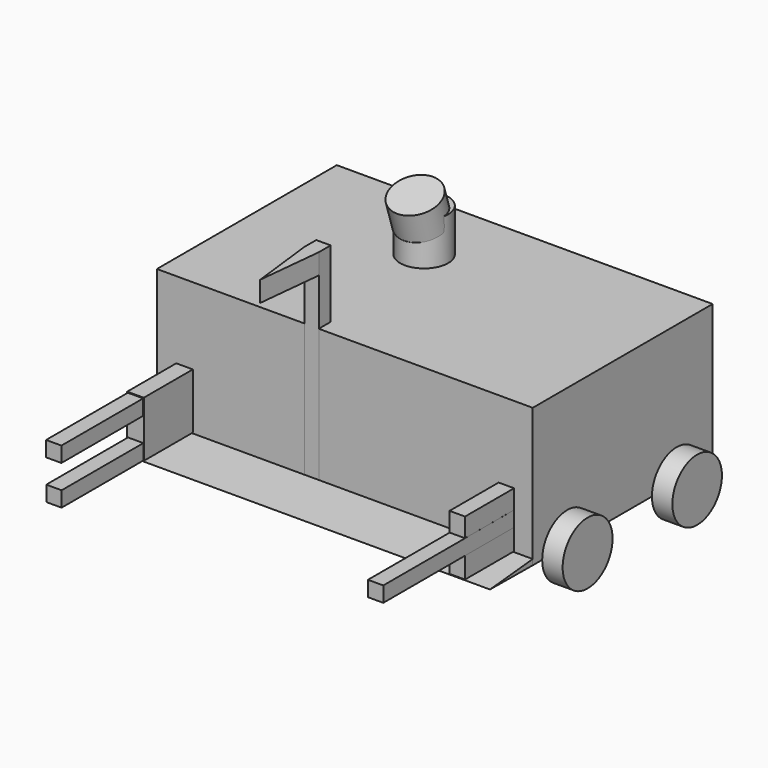
from build123d import *

# Parameters (mm, degrees)
F0_W      = 19.05
F0_H      = 19.05
F1_DEPTH  = 203.2
F2_W      = 20.5676518381
F2_H      = 69.0995454788
F3_DEPTH  = 76.2
F2_W_2    = 19.1925428808
F2_H_2    = 68.9241439104
F4_W      = 467.0027047396
F4_H      = 172.3322272301
F5_DEPTH  = 279.4
F6_R      = 38.6584580122
F7_DEPTH  = 19.05
F6_R_2    = 37.8719850625
F8_R      = 4.318122092
F9_DEPTH  = 26.924
F8_R_2    = 4.8859872563
F10_R     = 38.7883193787
F10_R_2   = 38.4875919081
F11_DEPTH = 25.4
F12_R     = 4.7009901189
F12_R_2   = 4.1671851321
F13_DEPTH = 24.13
F15_DEPTH = 464.82
F16_W     = 17.9072376341
F16_H     = 18.4862352908
F17_DEPTH = 230.632
F19_DEPTH = 25.4
F20_R     = 29.8192842647
F21_DEPTH = 53.34
F23_DEPTH = 61.976
F25_DEPTH = 33.02
F26_R     = 29.322274295
F27_DEPTH = 35.56
F28_R     = 29.0225579013
F29_DEPTH = 2.54
F30_R     = 23.7565214821
F31_DEPTH = 7.874
F32_R     = 28.9088352092
F33_DEPTH = 2.54
F34_R     = 42.3978860679
F35_DEPTH = 15.24
F36_R     = 32.2602250832
F37_DEPTH = 2.54
F38_R     = 23.6474446968
F39_DEPTH = 7.62
F40_R     = 31.7263717478
F41_DEPTH = 2.54


# Not quite as in the source:
# - a feature names something its author has since deleted; it is built from what else it names


with BuildPart() as f1:
    # F0 (on Front) → F1 (new body)
    with BuildSketch(Plane.XZ):
        with Locations((-148.8327021956, 35.0857683212)):
            Rectangle(F0_W, F0_H)
    extrude(amount=F1_DEPTH)


with BuildPart() as f1b:
    # F0 (on Front) → F1, piece 2 (new body)
    with BuildSketch(Plane.XZ):
        with Locations((-148.6062268972, -13.7355226338)):
            Rectangle(F0_W, F0_H)
    extrude(amount=F1_DEPTH)


with BuildPart() as f1c:
    # F0 (on Front) → F1, piece 3 (new body)
    with BuildSketch(Plane.XZ):
        with Locations((251.1326213121, 12.1724816259)):
            Rectangle(F0_W, F0_H)
    extrude(amount=F1_DEPTH)


with BuildPart() as f3:
    # F2 (on Front) → F3 (new body)
    with BuildSketch(Plane.XZ):
        with Locations((-148.8445419818, 11.0503323376)):
            Rectangle(F2_W, F2_H)
    extrude(amount=F3_DEPTH)


with BuildPart() as f3b:
    # F2 (on Front) → F3, piece 2 (new body)
    with BuildSketch(Plane.XZ):
        with Locations((251.0250490159, 10.9626315534)):
            Rectangle(F2_W_2, F2_H_2)
    extrude(amount=F3_DEPTH)


with BuildPart() as f5:
    # F4 (on Front) → F5 (new body)
    with BuildSketch(Plane.XZ):
        with Locations((50.3034517169, 54.7842234373)):
            Rectangle(F4_W, F4_H)
    extrude(amount=-F5_DEPTH)

    # F10 (on face) → F11 (join)
    with BuildSketch(Plane.YZ.offset(283.8048040867)):
        with Locations((53.4644015133, -31.3818901777)):
            Circle(F10_R)
        with Locations((223.617464304, -31.3818901777)):
            Circle(F10_R_2)
    extrude(amount=F11_DEPTH)

    # F12 (on face) → F13 (join)
    with BuildSketch(Plane.YZ.offset(283.8048040867)):
        with Locations((53.4644015133, -31.3818901777)):
            Circle(F12_R)
        with Locations((223.617464304, -31.3818901777)):
            Circle(F12_R_2)
    extrude(amount=-F13_DEPTH)

    # F20 (on face) → F21 (join)
    with BuildSketch(Plane.XY.offset(140.9503370523)):
        with Locations((0, 186.0438883305)):
            Circle(F20_R)
    extrude(amount=F21_DEPTH)

    # F22 (on face) → F23 (join)
    with BuildSketch(Plane.XY.offset(140.9503370523)):
        Polygon((15.8280599862, 196.6745853424), (-11.6345733404, 201.1040449142), (-11.6345733404, 171.869635582), (15.8280599862, 171.869635582), align=None)
    extrude(amount=F23_DEPTH)

    # F28 (on face) → F29 (join)
    with BuildSketch(Plane(origin=(0, 0, -31.3818901777), x_dir=(1, 0, 0), z_dir=(0, 0, -1))):
        with Locations((-63.1700456142, -252.9154121876)):
            Circle(F28_R)
    extrude(amount=F29_DEPTH)

    # F30 (on face) → F31 (join)
    with BuildSketch(Plane(origin=(0, 0, -33.9218901777), x_dir=(1, 0, 0), z_dir=(0, 0, -1))):
        with Locations((-63.1700456142, -252.9154121876)):
            Circle(F30_R)
    extrude(amount=F31_DEPTH)

    # F32 (on face) → F33 (join)
    with BuildSketch(Plane(origin=(0, 0, -41.7958901777), x_dir=(1, 0, 0), z_dir=(0, 0, -1))):
        with Locations((-63.1700456142, -252.9154121876)):
            Circle(F32_R)
    extrude(amount=F33_DEPTH)

    # F34 (on face) → F35 (join)
    with BuildSketch(Plane(origin=(0, 0, -31.3818901777), x_dir=(1, 0, 0), z_dir=(0, 0, -1))):
        with Locations((12.2496895492, -251.0914206505)):
            Circle(F34_R)
    extrude(amount=F35_DEPTH)

    # F36 (on face) → F37 (join)
    with BuildSketch(Plane(origin=(0, 0, -31.3818901777), x_dir=(1, 0, 0), z_dir=(0, 0, -1))):
        with Locations((-37.4250598252, -189.7709071636)):
            Circle(F36_R)
    extrude(amount=F37_DEPTH)

    # F38 (on face) → F39 (join)
    with BuildSketch(Plane(origin=(0, 0, -33.9218901777), x_dir=(1, 0, 0), z_dir=(0, 0, -1))):
        with Locations((-37.4250598252, -189.7709071636)):
            Circle(F38_R)
    extrude(amount=F39_DEPTH)

    # F40 (on face) → F41 (join)
    with BuildSketch(Plane(origin=(0, 0, -41.5418901777), x_dir=(1, 0, 0), z_dir=(0, 0, -1))):
        with Locations((-37.4250598252, -189.7709071636)):
            Circle(F40_R)
    extrude(amount=F41_DEPTH)


with BuildPart() as f7:
    # F6 (on face) → F7 (new body)
    with BuildSketch(Plane(origin=(-183.1979006529, 0, 0), x_dir=(0, -1, 0), z_dir=(-1, 0, 0))):
        with Locations((-54.0945269167, -31.3818901777)):
            Circle(F6_R)
    extrude(amount=F7_DEPTH)


with BuildPart() as f7b:
    # F6 (on face) → F7, piece 2 (new body)
    with BuildSketch(Plane(origin=(-183.1979006529, 0, 0), x_dir=(0, -1, 0), z_dir=(-1, 0, 0))):
        with Locations((-223.242148757, -31.3818901777)):
            Circle(F6_R_2)
    extrude(amount=F7_DEPTH)


with BuildPart() as f9:
    # F8 (on face) → F9 (new body)
    with BuildSketch(Plane(origin=(-183.1979006529, 0, 0), x_dir=(0, -1, 0), z_dir=(-1, 0, 0))):
        with Locations((-223.2621759176, -31.3818901777)):
            Circle(F8_R)
    extrude(amount=-F9_DEPTH)


with BuildPart() as f9b:
    # F8 (on face) → F9, piece 2 (new body)
    with BuildSketch(Plane(origin=(-183.1979006529, 0, 0), x_dir=(0, -1, 0), z_dir=(-1, 0, 0))):
        with Locations((-54.1642904282, -31.3818901777)):
            Circle(F8_R_2)
    extrude(amount=-F9_DEPTH)


with BuildPart() as f15:
    # F14 (on face) → F15 (new body)
    with BuildSketch(Plane.YZ.offset(283.8048040867)):
        Polygon((0, -31.3818901777), (0, -24.487003684), (-66.4077401161, -30.8189559728), align=None)
    extrude(amount=-F15_DEPTH)


with BuildPart() as f17:
    # F16 (on face) → F17 (new body)
    with BuildSketch(Plane(origin=(0, 0, -31.3818901777), x_dir=(1, 0, 0), z_dir=(0, 0, -1))):
        with Locations((8.953618817, -9.2431176454)):
            Rectangle(F16_W, F16_H)
    extrude(amount=-F17_DEPTH)

    # F18 (on face) → F19 (join)
    with BuildSketch(Plane.XY.offset(199.2501098223)):
        Polygon((17.9072376341, 18.4862352908), (0, 18.4862352908), (0, 0), (9.6268206835, -80.6094706059), (17.9072376341, 0), align=None)
    extrude(amount=F19_DEPTH)


with BuildPart() as f25:
    # F24 (on face) → F25 (new body)
    with BuildSketch(Plane.YZ.offset(15.8280599862)):
        Polygon((194.6656554937, 218.3648645878), (149.3803560734, 204.0061205626), (149.3803560734, 203.9490044117), align=None)
    extrude(amount=-F25_DEPTH)


with BuildPart() as f27:
    # F26 (on face) → F27 (new body)
    with BuildSketch(Plane(origin=(0, -45.1297047519, 142.3322394252), x_dir=(1, 0, 0), z_dir=(0, -0.30224368, 0.953230695))):
        with Locations((0, 227.807089798)):
            Circle(F26_R)
    extrude(amount=-F27_DEPTH)


solid = Compound([f1.part, f1b.part, f1c.part, f3.part, f3b.part, f5.part, f7.part, f7b.part, f9.part, f9b.part, f15.part, f17.part, f25.part, f27.part])
